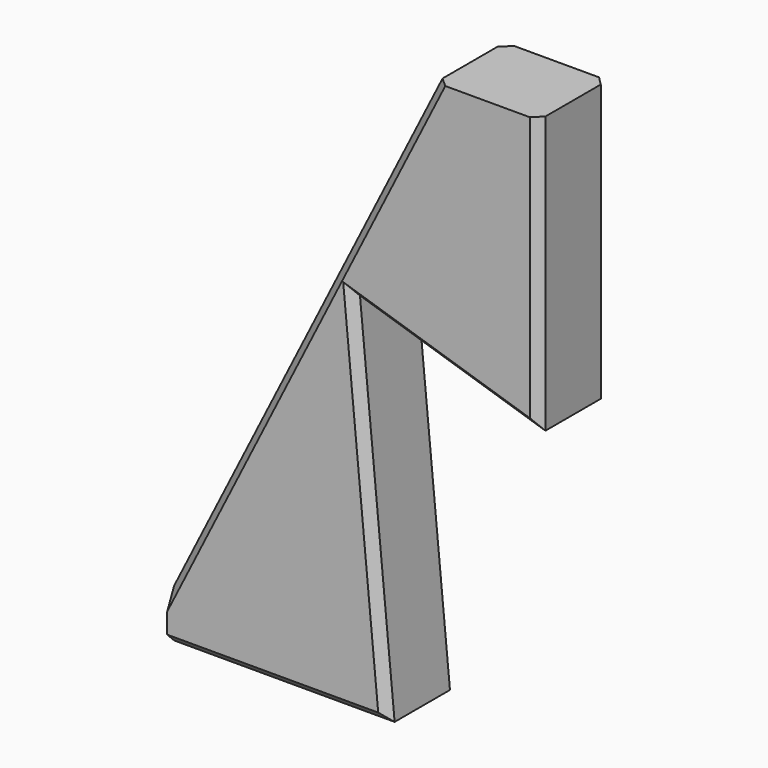
from build123d import *

# Parameters (mm, degrees)
F1_DEPTH = 10
F4_SIZE  = 1


# Not quite as in the source:
# - a feature of the source that left no trace in its solid (it failed there, or was rolled back) is left out


with BuildPart() as f1:
    # F0 (on Front) → F1 (new body)
    with BuildSketch(Plane.XZ):
        Polygon((0, -25.5473433032), (0, -31.1332004264), (25.5, -31.1332004264), (21.4898194077, 10.9762813041), (42.9413538213, 4.1879331029), (42.9413538213, 36.1879331029), (31.0413538213, 36.1879331029), align=None)
    extrude(amount=F1_DEPTH)

    # F4
    f4_edges = [f1.edges().sort_by_distance(p)[0] for p in [
        (23.49491, 0, -10.07846),
        (32.215587, 0, 7.582107),
        (42.941354, 0, 20.187933),
        (15.520677, 0, 5.320295),
        (23.49491, -10, -10.07846),
        (32.215587, -10, 7.582107),
        (42.941354, -10, 20.187933),
        (15.520677, -10, 5.320295),
        (12.75, 0, -31.1332),
        (12.75, -10, -31.1332),
    ]]
    chamfer(f4_edges, length=F4_SIZE)


solid = f1.part
